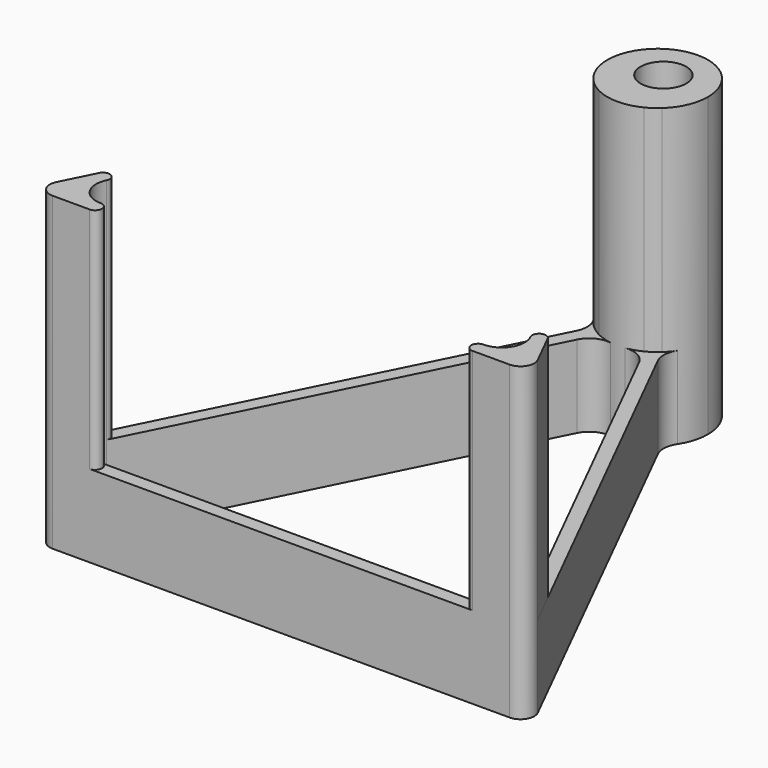
from build123d import *

# Parameters (mm, degrees)
F1_DEPTH    = 65
F2_DEPTH    = 18
F3_DEPTH    = 65
F4_R        = 5
F5_T1_DEPTH = 18
F7_DEPTH    = 50
F8_R        = 5
F8_R_2      = 2
F9_DEPTH    = 63


# Not quite as in the source:
# - a fillet or chamfer that OpenCascade refuses, or shapes differently, is made with other operations: its cross-section is extruded or revolved along the edge and cut away or added


with BuildPart() as f1:
    # F0 (on Top) → F1 (new body)
    with BuildSketch(Plane.XY):
        with BuildLine():
            ThreePointArc((11, 100), (-4.4397297556, 110.0642336865), (-7.4161453995, 91.8759131335))
            Line((-7.4161453995, 91.8759131335), (-4.039885348, 98.6284332366))
            ThreePointArc((-4.039885348, 98.6284332366), (-1.5492858452, 106.3284184683), (5, 101.5745028853))
            ThreePointArc((5, 101.5745028853), (4.753915583, 100.0252170402), (4.039885348, 98.6284332366))
            Line((4.039885348, 98.6284332366), (7.4161453995, 91.8759131335))
            ThreePointArc((7.4161453995, 91.8759131335), (10.0642336865, 95.5602702444), (11, 100))
        make_face()
        with BuildLine():
            Line((-1.5839824005, 96.8320351991), (-4.9193495505, 90.161300899))
            ThreePointArc((-4.9193495505, 90.161300899), (0, 89), (4.9193495505, 90.161300899))
            Line((4.9193495505, 90.161300899), (1.5839824005, 96.8320351991))
            ThreePointArc((1.5839824005, 96.8320351991), (0, 96.5745028853), (-1.5839824005, 96.8320351991))
        make_face()
        with BuildLine():
            ThreePointArc((-7.4161453995, 91.8759131335), (-6.227044459, 90.9322595259), (-4.9193495505, 90.161300899))
            Line((-4.9193495505, 90.161300899), (-1.5839824005, 96.8320351991))
            ThreePointArc((-1.5839824005, 96.8320351991), (-2.9519033843, 97.5388782237), (-4.039885348, 98.6284332366))
            Line((-4.039885348, 98.6284332366), (-7.4161453995, 91.8759131335))
        make_face()
        with BuildLine():
            Line((1.5839824005, 96.8320351991), (4.9193495505, 90.161300899))
            ThreePointArc((4.9193495505, 90.161300899), (6.227044459, 90.9322595259), (7.4161453995, 91.8759131335))
            Line((7.4161453995, 91.8759131335), (4.039885348, 98.6284332366))
            ThreePointArc((4.039885348, 98.6284332366), (2.9519033843, 97.5388782237), (1.5839824005, 96.8320351991))
        make_face()
        with BuildLine():
            Line((-0.2073593004, 99.5852813993), (-1.5839824005, 96.8320351991))
            ThreePointArc((-1.5839824005, 96.8320351991), (0, 96.5745028853), (1.5839824005, 96.8320351991))
            Line((1.5839824005, 96.8320351991), (0.2073593004, 99.5852813993))
            ThreePointArc((0.2073593004, 99.5852813993), (0, 99.5745028853), (-0.2073593004, 99.5852813993))
        make_face()
        with BuildLine():
            ThreePointArc((-4.039885348, 98.6284332366), (-2.9519033843, 97.5388782237), (-1.5839824005, 96.8320351991))
            Line((-1.5839824005, 96.8320351991), (-0.2073593004, 99.5852813993))
            ThreePointArc((-0.2073593004, 99.5852813993), (-1.7280798318, 100.567656276), (-1.8327895721, 102.3750541855))
            ThreePointArc((-1.8327895721, 102.3750541855), (-2.3164003238, 101.9063812682), (-2.683281573, 101.3416407865))
            Line((-2.683281573, 101.3416407865), (-4.039885348, 98.6284332366))
        make_face()
        with BuildLine():
            ThreePointArc((5, 101.5745028853), (-1.5492858452, 106.3284184683), (-4.039885348, 98.6284332366))
            Line((-4.039885348, 98.6284332366), (-2.683281573, 101.3416407865))
            ThreePointArc((-2.683281573, 101.3416407865), (-2.3164003238, 101.9063812682), (-1.8327895721, 102.3750541855))
            ThreePointArc((-1.8327895721, 102.3750541855), (0, 103.5745028853), (1.8327895721, 102.3750541855))
            ThreePointArc((1.8327895721, 102.3750541855), (2.3164003238, 101.9063812682), (2.683281573, 101.3416407865))
            Line((2.683281573, 101.3416407865), (4.039885348, 98.6284332366))
            ThreePointArc((4.039885348, 98.6284332366), (4.753915583, 100.0252170402), (5, 101.5745028853))
        make_face()
        with BuildLine():
            Line((0.2073593004, 99.5852813993), (1.5839824005, 96.8320351991))
            ThreePointArc((1.5839824005, 96.8320351991), (2.9519033843, 97.5388782237), (4.039885348, 98.6284332366))
            Line((4.039885348, 98.6284332366), (2.683281573, 101.3416407865))
            ThreePointArc((2.683281573, 101.3416407865), (2.3164003238, 101.9063812682), (1.8327895721, 102.3750541855))
            ThreePointArc((1.8327895721, 102.3750541855), (1.9577511517, 101.9834166022), (2, 101.5745028853))
            ThreePointArc((2, 101.5745028853), (1.4857184459, 100.2356075572), (0.2073593004, 99.5852813993))
        make_face()
        with BuildLine():
            ThreePointArc((-1.8327895721, 102.3750541855), (-1.7280798318, 100.567656276), (-0.2073593004, 99.5852813993))
            Line((-0.2073593004, 99.5852813993), (0, 100))
            Line((0, 100), (0.2073593004, 99.5852813993))
            ThreePointArc((0.2073593004, 99.5852813993), (1.4857184459, 100.2356075572), (2, 101.5745028853))
            ThreePointArc((2, 101.5745028853), (1.9577511517, 101.9834166022), (1.8327895721, 102.3750541855))
            ThreePointArc((1.8327895721, 102.3750541855), (0, 103), (-1.8327895721, 102.3750541855))
        make_face()
        with BuildLine():
            Line((0, 100), (-0.2073593004, 99.5852813993))
            ThreePointArc((-0.2073593004, 99.5852813993), (0, 99.5745028853), (0.2073593004, 99.5852813993))
            Line((0.2073593004, 99.5852813993), (0, 100))
        make_face()
        with BuildLine():
            ThreePointArc((1.8327895721, 102.3750541855), (0, 103.5745028853), (-1.8327895721, 102.3750541855))
            ThreePointArc((-1.8327895721, 102.3750541855), (0, 103), (1.8327895721, 102.3750541855))
        make_face()
    extrude(amount=F1_DEPTH)

    # F0 (on Top) → F2 (join)
    with BuildSketch(Plane.XY):
        with BuildLine():
            Line((50, 0), (-50, 0))
            Line((-50, 0), (-4.9193495505, 90.161300899))
            ThreePointArc((-4.9193495505, 90.161300899), (-6.227044459, 90.9322595259), (-7.4161453995, 91.8759131335))
            Line((-7.4161453995, 91.8759131335), (-52.683281573, 1.3416407865))
            ThreePointArc((-52.683281573, 1.3416407865), (-52.5519524251, -1.5771933364), (-50, -3))
            Line((-50, -3), (50, -3))
            ThreePointArc((50, -3), (52.5519524251, -1.5771933364), (52.683281573, 1.3416407865))
            Line((52.683281573, 1.3416407865), (7.4161453995, 91.8759131335))
            ThreePointArc((7.4161453995, 91.8759131335), (6.227044459, 90.9322595259), (4.9193495505, 90.161300899))
            Line((4.9193495505, 90.161300899), (50, 0))
        make_face()
    extrude(amount=F2_DEPTH)

    # F0 (on Top) → F3 (cut)
    with BuildSketch(Plane.XY):
        with BuildLine():
            ThreePointArc((-1.8327895721, 102.3750541855), (-1.7280798318, 100.567656276), (-0.2073593004, 99.5852813993))
            Line((-0.2073593004, 99.5852813993), (0, 100))
            Line((0, 100), (0.2073593004, 99.5852813993))
            ThreePointArc((0.2073593004, 99.5852813993), (1.4857184459, 100.2356075572), (2, 101.5745028853))
            ThreePointArc((2, 101.5745028853), (1.9577511517, 101.9834166022), (1.8327895721, 102.3750541855))
            ThreePointArc((1.8327895721, 102.3750541855), (0, 103), (-1.8327895721, 102.3750541855))
        make_face()
        with BuildLine():
            ThreePointArc((1.8327895721, 102.3750541855), (0, 103.5745028853), (-1.8327895721, 102.3750541855))
            ThreePointArc((-1.8327895721, 102.3750541855), (0, 103), (1.8327895721, 102.3750541855))
        make_face()
        with BuildLine():
            Line((0, 100), (-0.2073593004, 99.5852813993))
            ThreePointArc((-0.2073593004, 99.5852813993), (0, 99.5745028853), (0.2073593004, 99.5852813993))
            Line((0.2073593004, 99.5852813993), (0, 100))
        make_face()
    extrude(amount=F3_DEPTH, mode=Mode.SUBTRACT)

    # F4
    f4_edges = [f1.edges().sort_by_distance(p)[0] for p in [
        (50, 0, 9),
    ]]
    fillet(f4_edges, radius=F4_R)

    # F5: fillet of radius 5 on 5 edges, made by hand

    # F5_s2 → F5_t1 (join)
    with BuildSketch(Plane.XY):
        with BuildLine():
            ThreePointArc((-41.9098300563, 0), (-46.163084098, 2.3713444394), (-46.3819660113, 7.2360679775))
            Line((-46.3819660113, 7.2360679775), (-50, 0))
            Line((-50, 0), (-41.9098300563, 0))
        make_face()
        with BuildLine():
            ThreePointArc((6.7970581872, 86.4058836256), (4.6367553585, 88.6032598618), (1.5983840346, 89.1167482581))
            ThreePointArc((1.5983840346, 89.1167482581), (3.3004522912, 89.5068110341), (4.9193495505, 90.161300899))
            Line((4.9193495505, 90.161300899), (6.7970581872, 86.4058836256))
        make_face()
        with BuildLine():
            ThreePointArc((9.1796312313, 93.9391114136), (8.361173547, 91.4837383605), (8.8800549269, 88.9480940786))
            Line((8.8800549269, 88.9480940786), (7.4161453995, 91.8759131335))
            ThreePointArc((7.4161453995, 91.8759131335), (8.3617669951, 92.8529129906), (9.1796312313, 93.9391114136))
        make_face()
        with BuildLine():
            ThreePointArc((-9.1796312313, 93.9391114136), (-8.361173547, 91.4837383605), (-8.8800549269, 88.9480940786))
            Line((-8.8800549269, 88.9480940786), (-7.4161453995, 91.8759131335))
            ThreePointArc((-7.4161453995, 91.8759131335), (-8.3617669951, 92.8529129906), (-9.1796312313, 93.9391114136))
        make_face()
        with BuildLine():
            ThreePointArc((-1.5983840346, 89.1167482581), (-4.6367553585, 88.6032598618), (-6.7970581872, 86.4058836256))
            Line((-6.7970581872, 86.4058836256), (-4.9193495505, 90.161300899))
            ThreePointArc((-4.9193495505, 90.161300899), (-3.3004522912, 89.5068110341), (-1.5983840346, 89.1167482581))
        make_face()
    extrude(amount=F5_T1_DEPTH)

    # F6 (on face) → F7 (join)
    with BuildSketch(Plane.XY.offset(18)):
        with BuildLine():
            ThreePointArc((41.9098300563, 0), (40.4098300563, -1.5), (41.9098300563, -3))
            Line((41.9098300563, -3), (50, -3))
            ThreePointArc((50, -3), (52.5519524251, -1.5771933364), (52.683281573, 1.3416407865))
            Line((52.683281573, 1.3416407865), (49.0652475842, 8.577708764))
            ThreePointArc((49.0652475842, 8.577708764), (47.0527864045, 9.2485291572), (46.3819660113, 7.2360679775))
            ThreePointArc((46.3819660113, 7.2360679775), (46.163084098, 2.3713444394), (41.9098300563, 0))
        make_face()
        with BuildLine():
            Line((-50, -3), (-41.9098300563, -3))
            ThreePointArc((-41.9098300563, -3), (-40.4098300563, -1.5), (-41.9098300563, 0))
            ThreePointArc((-41.9098300563, 0), (-46.163084098, 2.3713444394), (-46.3819660113, 7.2360679775))
            ThreePointArc((-46.3819660113, 7.2360679775), (-47.0527864045, 9.2485291572), (-49.0652475842, 8.577708764))
            Line((-49.0652475842, 8.577708764), (-52.683281573, 1.3416407865))
            ThreePointArc((-52.683281573, 1.3416407865), (-52.5519524251, -1.5771933364), (-50, -3))
        make_face()
    extrude(amount=F7_DEPTH)

    # F8 (on face) → F9 (cut)
    with BuildSketch(Plane.XY.offset(65)):
        with Locations((0, 101.5745028853)):
            Circle(F8_R)
        with Locations((0, 101.5745028853)):
            Circle(F8_R_2, mode=Mode.SUBTRACT)
    extrude(amount=-F9_DEPTH, mode=Mode.SUBTRACT)


solid = f1.part
